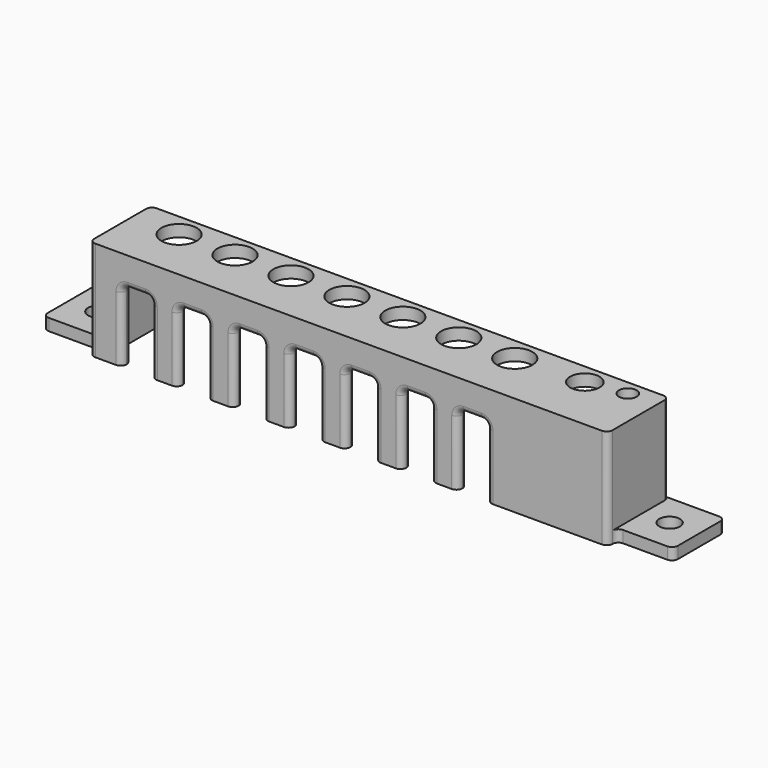
from build123d import *

# Parameters (mm, degrees)
F0_W     = 9.5
F0_H     = 11
F0_R     = 1.75
F1_DEPTH = 2
F2_DEPTH = 17
F0_W_2   = 84
F3_DEPTH = 17
F4_DEPTH = 15
F6_DEPTH = 13.001
F7_R     = 3
F7_R_2   = 2.5
F7_R_3   = 1.5
F8_DEPTH = 25
F9_R     = 0.99999
F10_R    = 0.99999


# Not quite as in the source:
# - a fillet or chamfer is up to 0.001 mm smaller than in the source, because OpenCascade refuses the exact size


with BuildPart() as f1:
    # F0 (on Top) → F1 (new body)
    with BuildSketch(Plane.XY):
        with Locations((46.75, 17.5)):
            Rectangle(F0_W, F0_H)
        with Locations((46.5, 17.5)):
            Circle(F0_R, mode=Mode.SUBTRACT)
    extrude(amount=F1_DEPTH)



with BuildPart() as f1b:
    # F0 (on Top) → F1, piece 2 (new body)
    with BuildSketch(Plane.XY):
        with Locations((-50.75, 17.5)):
            Rectangle(F0_W, F0_H)
        with Locations((-50.5, 17.5)):
            Circle(F0_R, mode=Mode.SUBTRACT)
    extrude(amount=F1_DEPTH)


with BuildPart() as f1_1:
    add(f1.part)

    add(f1b.part)  # F2 merges F1b
    # F0 (on Top) → F2 (join)
    with BuildSketch(Plane.XY):
        Polygon((-44, 23), (-46, 23), (-46, 12), (-46, 10), (42, 10), (42, 12), (42, 23), (40, 23), (40, 12), (-44, 12), align=None)
    extrude(amount=F2_DEPTH)

    # F0 (on Top) → F3 (join)
    with BuildSketch(Plane.XY):
        with Locations((-2, 17.5)):
            Rectangle(F0_W_2, F0_H)
    extrude(amount=F3_DEPTH)

    # F0 (on Top) → F4 (cut)
    with BuildSketch(Plane.XY):
        with Locations((-2, 17.5)):
            Rectangle(F0_W_2, F0_H)
    extrude(amount=F4_DEPTH, mode=Mode.SUBTRACT)

    # F5 (on face) → F6 (cut, through all)
    with BuildSketch(Plane.XZ.offset(-10)):
        with BuildLine():
            Line((-36.5, 12), (-39.5, 12))
            ThreePointArc((-39.5, 12), (-40.2071067812, 11.7071067812), (-40.5, 11))
            Line((-40.5, 11), (-40.5, 0))
            Line((-40.5, 0), (-35.5, 0))
            Line((-35.5, 0), (-35.5, 11))
            ThreePointArc((-35.5, 11), (-35.7928932188, 11.7071067812), (-36.5, 12))
        make_face()
        with BuildLine():
            Line((-31, 11), (-31, 0))
            Line((-31, 0), (-26, 0))
            Line((-26, 0), (-26, 11))
            ThreePointArc((-26, 11), (-26.2928932188, 11.7071067812), (-27, 12))
            Line((-27, 12), (-30, 12))
            ThreePointArc((-30, 12), (-30.7071067812, 11.7071067812), (-31, 11))
        make_face()
        with BuildLine():
            Line((-21.5, 11), (-21.5, 0))
            Line((-21.5, 0), (-16.5, 0))
            Line((-16.5, 0), (-16.5, 11))
            ThreePointArc((-16.5, 11), (-16.7928932188, 11.7071067812), (-17.5, 12))
            Line((-17.5, 12), (-20.5, 12))
            ThreePointArc((-20.5, 12), (-21.2071067812, 11.7071067812), (-21.5, 11))
        make_face()
        with BuildLine():
            Line((-12, 11), (-12, 0))
            Line((-12, 0), (-7, 0))
            Line((-7, 0), (-7, 11))
            ThreePointArc((-7, 11), (-7.2928932188, 11.7071067812), (-8, 12))
            Line((-8, 12), (-11, 12))
            ThreePointArc((-11, 12), (-11.7071067812, 11.7071067812), (-12, 11))
        make_face()
        with BuildLine():
            Line((-2.5, 11), (-2.5, 0))
            Line((-2.5, 0), (2.5, 0))
            Line((2.5, 0), (2.5, 11))
            ThreePointArc((2.5, 11), (2.2071067812, 11.7071067812), (1.5, 12))
            Line((1.5, 12), (-1.5, 12))
            ThreePointArc((-1.5, 12), (-2.2071067812, 11.7071067812), (-2.5, 11))
        make_face()
        with BuildLine():
            Line((7, 0), (12, 0))
            Line((12, 0), (12, 11))
            ThreePointArc((12, 11), (11.7071067812, 11.7071067812), (11, 12))
            Line((11, 12), (8, 12))
            ThreePointArc((8, 12), (7.2928932188, 11.7071067812), (7, 11))
            Line((7, 11), (7, 0))
        make_face()
        with BuildLine():
            Line((16.5, 0), (21.5, 0))
            Line((21.5, 0), (21.5, 11))
            ThreePointArc((21.5, 11), (21.2071067812, 11.7071067812), (20.5, 12))
            Line((20.5, 12), (17.5, 12))
            ThreePointArc((17.5, 12), (16.7928932188, 11.7071067812), (16.5, 11))
            Line((16.5, 11), (16.5, 0))
        make_face()
    extrude(amount=-F6_DEPTH, mode=Mode.SUBTRACT)

    # F7 (on face) → F8 (cut)
    with BuildSketch(Plane.XY.offset(17)):
        with Locations((-38, 19)):
            Circle(F7_R)
        with Locations((-28.5, 19)):
            Circle(F7_R)
        with Locations((-19, 19)):
            Circle(F7_R)
        with Locations((-9.5, 19)):
            Circle(F7_R)
        with Locations((9.5, 19)):
            Circle(F7_R)
        with Locations((19, 19)):
            Circle(F7_R)
        with Locations((30.5, 19.5)):
            Circle(F7_R_2)
        with Locations((37, 20.5)):
            Circle(F7_R_3)
        with Locations((0, 19)):
            Circle(F7_R)
    extrude(amount=-F8_DEPTH, mode=Mode.SUBTRACT)

    # F9 (radius 1 in the source; OpenCascade refuses exactly that, so slightly less here)
    f9_edges = [f1_1.edges().sort_by_distance(p)[0] for p in [
        (-40.5, 10, 5.5),
        (-40.5, 12, 5.5),
        (-31, 10, 5.5),
        (-31, 12, 5.5),
        (-21.5, 10, 5.5),
        (-21.5, 12, 5.5),
        (-12, 10, 5.5),
        (-12, 12, 5.5),
        (-2.5, 10, 5.5),
        (-2.5, 12, 5.5),
        (7, 10, 5.5),
        (7, 12, 5.5),
        (16.5, 10, 5.5),
        (16.5, 12, 5.5),
    ]]
    fillet(f9_edges, radius=F9_R)

    # F10 (radius 1 in the source; OpenCascade refuses exactly that, so slightly less here)
    f10_edges = [f1_1.edges().sort_by_distance(p)[0] for p in [
        (-46, 10, 8.5),
        (-46, 12, 1),
        (-55.5, 12, 1),
        (-55.5, 23, 1),
        (-46, 23, 9.5),
        (-44, 23, 7.5),
        (40, 23, 7.5),
        (42, 23, 9.5),
        (51.5, 23, 1),
        (51.5, 12, 1),
        (42, 10, 8.5),
        (42, 12, 1),
        (40, 12, 7.5),
        (-44, 12, 7.5),
    ]]
    fillet(f10_edges, radius=F10_R)


solid = f1_1.part
